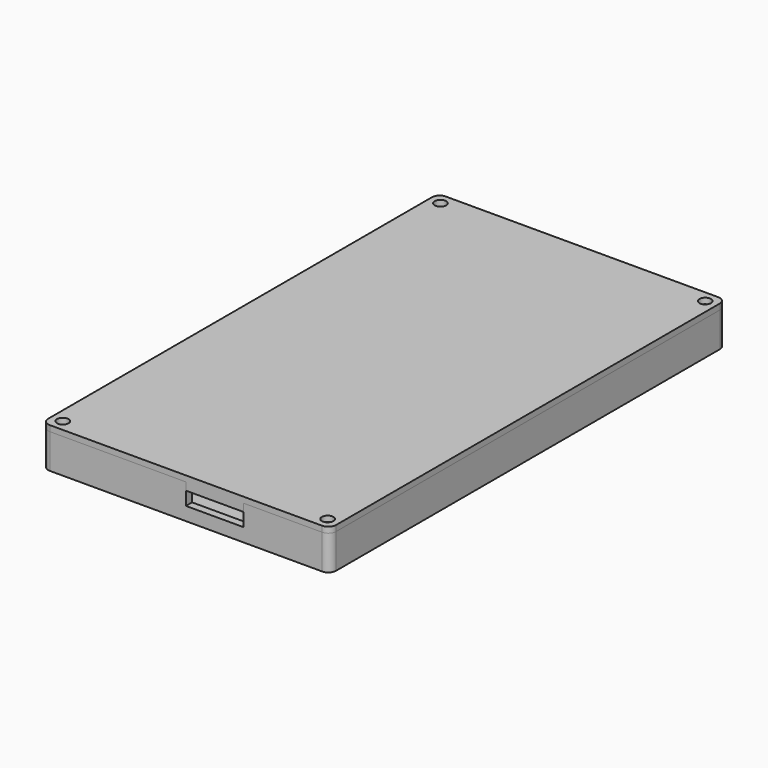
from build123d import *

# Parameters (mm, degrees)
F0_R     = 1.25
F0_W     = 15
F0_H     = 2
F1_DEPTH = 1.5
F2_DEPTH = 7.5
F3_R     = 2
F4_DEPTH = 2
F5_R     = 1.5
F5_W     = 15
F5_H     = 2
F6_DEPTH = 1.5
F7_R     = 2
F8_DEPTH = 2


# Not quite as in the source:
# - a feature names something its author has since deleted; it is built from what else it names


with BuildPart() as f1:
    # F0 (on Top) → F1 (new body)
    with BuildSketch(Plane.XY):
        Polygon((-35.5, -50.5), (-35.5, 50.5), (-31.5, 50.5), (-31.5, 54.5), (31.5, 54.5), (31.5, 50.5), (35.5, 50.5), (35.5, -50.5), (31.5, -50.5), (31.5, -70.5), (15, -70.5), (15, -72.5), (37.5, -72.5), (37.5, -56.5), (37.5, 56.5), (-37.5, 56.5), (-37.5, -56.5), (-37.5, -72.5), (0, -72.5), (0, -70.5), (-31.5, -70.5), (-31.5, -50.5), align=None)
        with Locations((-34.5, -69.5)):
            Circle(F0_R, mode=Mode.SUBTRACT)
        with Locations((34.5, -69.5)):
            Circle(F0_R, mode=Mode.SUBTRACT)
        with Locations((-34.5, 53.5)):
            Circle(F0_R, mode=Mode.SUBTRACT)
        with Locations((34.5, 53.5)):
            Circle(F0_R, mode=Mode.SUBTRACT)
        Polygon((-31.5, 50.5), (-35.5, 50.5), (-35.5, -50.5), (-31.5, -50.5), (-31.5, -70.5), (0, -70.5), (15, -70.5), (31.5, -70.5), (31.5, -50.5), (35.5, -50.5), (35.5, 50.5), (31.5, 50.5), (31.5, 54.5), (-31.5, 54.5), align=None)
        with Locations((7.5, -71.5)):
            Rectangle(F0_W, F0_H)
    extrude(amount=-F1_DEPTH)

    # F0 (on Top) → F2 (join)
    with BuildSketch(Plane.XY):
        Polygon((-35.5, -50.5), (-35.5, 50.5), (-31.5, 50.5), (-31.5, 54.5), (31.5, 54.5), (31.5, 50.5), (35.5, 50.5), (35.5, -50.5), (31.5, -50.5), (31.5, -70.5), (15, -70.5), (15, -72.5), (37.5, -72.5), (37.5, -56.5), (37.5, 56.5), (-37.5, 56.5), (-37.5, -56.5), (-37.5, -72.5), (0, -72.5), (0, -70.5), (-31.5, -70.5), (-31.5, -50.5), align=None)
        with Locations((-34.5, -69.5)):
            Circle(F0_R, mode=Mode.SUBTRACT)
        with Locations((34.5, -69.5)):
            Circle(F0_R, mode=Mode.SUBTRACT)
        with Locations((-34.5, 53.5)):
            Circle(F0_R, mode=Mode.SUBTRACT)
        with Locations((34.5, 53.5)):
            Circle(F0_R, mode=Mode.SUBTRACT)
    extrude(amount=F2_DEPTH)

    # F3
    f3_edges = [f1.edges().sort_by_distance(p)[0] for p in [
        (37.5, 56.5, 3),
        (-37.5, 56.5, 3),
        (31.5, -50.5, 3.75),
        (-31.5, 50.5, 3.75),
        (31.5, 50.5, 3.75),
        (-31.5, -50.5, 3.75),
        (37.5, -72.5, 3),
        (-37.5, -72.5, 3),
        (-31.5, -70.5, 3.75),
    ]]
    fillet(f3_edges, radius=F3_R)

    # F0 (on Top) → F4 (join)
    with BuildSketch(Plane.XY):
        with Locations((7.5, -71.5)):
            Rectangle(F0_W, F0_H)
    extrude(amount=F4_DEPTH)


with BuildPart() as f6:
    # F5 (on face) → F6 (new body)
    with BuildSketch(Plane.XY.offset(7.5)):
        Polygon((37.5, -72.5), (37.5, 56.5), (-37.5, 56.5), (-37.5, -72.5), (0, -72.5), (0, -70.5), (15, -70.5), (15, -72.5), align=None)
        with Locations((-34.5, -69.5)):
            Circle(F5_R, mode=Mode.SUBTRACT)
        with Locations((34.5, -69.5)):
            Circle(F5_R, mode=Mode.SUBTRACT)
        with Locations((-34.5, 53.5)):
            Circle(F5_R, mode=Mode.SUBTRACT)
        with Locations((34.5, 53.5)):
            Circle(F5_R, mode=Mode.SUBTRACT)
        with Locations((7.5, -71.5)):
            Rectangle(F5_W, F5_H)
    extrude(amount=F6_DEPTH)

    # F7
    f7_edges = [f6.edges().sort_by_distance(p)[0] for p in [
        (-37.5, 56.5, 8.25),
        (37.5, 56.5, 8.25),
        (-37.5, -72.5, 8.25),
        (37.5, -72.5, 8.25),
    ]]
    fillet(f7_edges, radius=F7_R)

    # F5 (on face) → F8 (join)
    with BuildSketch(Plane.XY.offset(7.5)):
        with Locations((7.5, -71.5)):
            Rectangle(F5_W, F5_H)
    extrude(amount=-F8_DEPTH)


solid = Compound([f1.part, f6.part])
